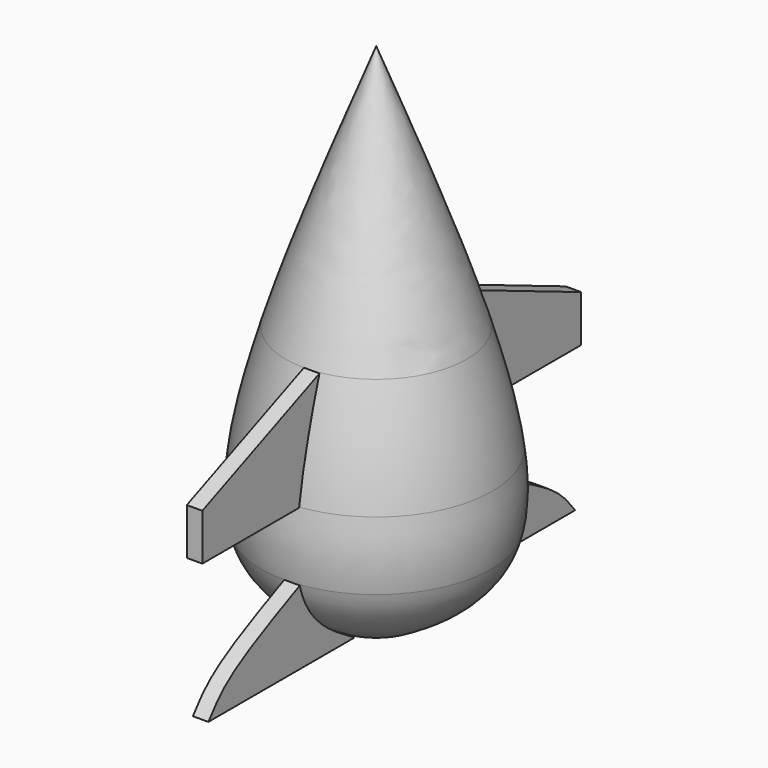
from build123d import *

# Parameters (mm, degrees)
F4_DEPTH = 5
F6_DEPTH = 5


# Not quite as in the source:
# - a feature of the source that left no trace in its solid (it failed there, or was rolled back) is left out
# - the program builds the solid bodies; features that only make, move or delete a surface that nothing else refers to are left out


with BuildPart() as f1:
    # F0 (on Right) → F1 (revolve)
    with BuildSketch(Plane.YZ):
        with BuildLine():
            Line((0, 160), (0, 0))
            Line((0, 0), (15, 0))
            add(Edge.make_bspline(
                [(15, 0), (24.4865858745, 5.6652130966), (33.9731717491, 11.3304261932), (37.0251424611, 23.7176921219)],
                knots=[0, 0, 0, 0, 0.3237492422, 0.3237492422, 0.3237492422, 0.3237492422], degree=3))
            add(Edge.make_bspline(
                [(37.0251424611, 23.7176921219), (38.4909770242, 29.667186483), (38.4724771265, 37.1673213121), (37.3109436119, 45.8615496754)],
                knots=[0.3237492422, 0.3237492422, 0.3237492422, 0.3237492422, 0.4792431423, 0.4792431423, 0.4792431423, 0.4792431423], degree=3))
            add(Edge.make_bspline(
                [(37.3109436119, 45.8615496754), (35.9546245135, 56.0137732894), (33.0397607, 67.794162637), (29.1097623357, 80.6350331336)],
                knots=[0.4792431423, 0.4792431423, 0.4792431423, 0.4792431423, 0.6608128894, 0.6608128894, 0.6608128894, 0.6608128894], degree=3))
            add(Edge.make_bspline(
                [(29.1097623357, 80.6350331336), (21.7682045505, 104.6228275357), (10.8841022753, 132.3114137679), (0, 160)],
                knots=[0.6608128894, 0.6608128894, 0.6608128894, 0.6608128894, 1, 1, 1, 1], degree=3))
        make_face()
    revolve(axis=Axis((0, 0, 80), (0, 0, 1)))


with BuildPart() as f4:
    # F0 (on Right) → F4 (new body)
    with BuildSketch(Plane.YZ):
        with BuildLine():
            Line((76.2734785671, 60.8615496754), (29.1097623357, 80.6350331336))
            add(Edge.make_bspline(
                [(37.3109436119, 45.8615496754), (35.9546245135, 56.0137732894), (33.0397607, 67.794162637), (29.1097623357, 80.6350331336)],
                knots=[0.4792431423, 0.4792431423, 0.4792431423, 0.4792431423, 0.6608128894, 0.6608128894, 0.6608128894, 0.6608128894], degree=3))
            Line((37.3109436119, 45.8615496754), (76.2734785671, 45.8615496754))
            Line((76.2734785671, 45.8615496754), (76.2734785671, 60.8615496754))
        make_face()
    extrude(amount=F4_DEPTH)


with BuildPart() as f5_1:
    # F5: instance of F4
    add(f4.part.mirror(Plane.XZ))


with BuildPart() as f6:
    # F0 (on Right) → F6 (new body)
    with BuildSketch(Plane.YZ):
        with BuildLine():
            add(Edge.make_bspline(
                [(15, 0), (24.4865858745, 5.6652130966), (33.9731717491, 11.3304261932), (37.0251424611, 23.7176921219)],
                knots=[0, 0, 0, 0, 0.3237492422, 0.3237492422, 0.3237492422, 0.3237492422], degree=3))
            Line((15, 0), (73.8379135728, 0))
            add(Edge.make_bspline(
                [(73.8379135728, 0), (71.6348183096, 2.8776720373), (65.8334199202, 10.4554296596), (48.053249542, 18.640760647), (37.0251424611, 23.7176921219)],
                knots=[0, 0, 0, 0, 0.379752452, 1, 1, 1, 1], degree=3))
        make_face()
    extrude(amount=F6_DEPTH)


with BuildPart() as f7_1:
    # F7: instance of F6
    add(f6.part.mirror(Plane.XZ))


solid = Compound([f1.part, f4.part, f5_1.part, f6.part, f7_1.part])
